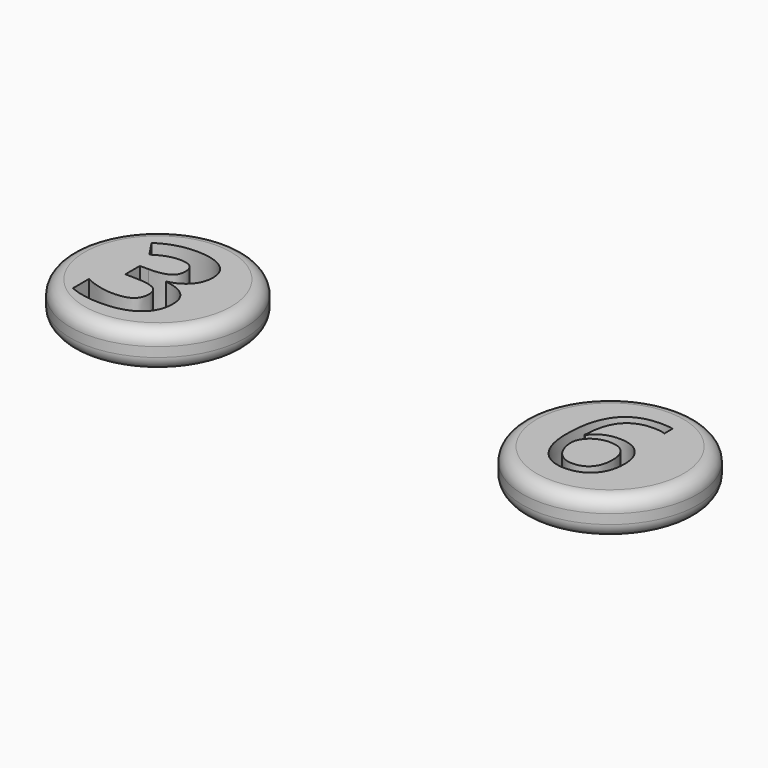
from build123d import *

# Parameters (mm, degrees)
F0_R         = 15.498811994
F1_DEPTH     = 6.604
F2_R         = 2.4528409794
F4_TEXT_SIZE = 27.8857070194
F5_DEPTH     = 25.4
F7_TEXT_SIZE = 25.6220861855
F8_DEPTH     = 25.4


# Not quite as in the source:
# - Text() gives the source's letters only with a copy of the font that has no kerning and outlines rounded to 1/6400 em; it was checked with that copy


with BuildPart() as f1:
    # F0 (on Top) → F1 (new body)
    with BuildSketch(Plane.XY):
        with Locations((-40.1489026845, 21.7293333262)):
            Circle(F0_R)
    extrude(amount=F1_DEPTH)

    # F2
    f2_edges = [f1.edges().sort_by_distance(p)[0] for p in [
        (-55.647715, 21.729333, 0),
        (-55.647715, 21.729333, 6.604),
    ]]
    fillet(f2_edges, radius=F2_R)


with BuildPart() as f3_1:
    # F3: instance of F1
    add(f1.part.mirror(Plane.YZ))

    # F7 (on face) → F8 (cut)
    with BuildSketch(Plane.XY.offset(6.604)):
        with Locations((31.6101685166, 12.9549875855)):
            Text('6', F7_TEXT_SIZE, font='Open Sans', text_align=(TextAlign.LEFT, TextAlign.BOTTOM))
    extrude(amount=-F8_DEPTH, mode=Mode.SUBTRACT)


with BuildPart() as f1_1:
    add(f1.part)

    # F4 (on face) → F5 (cut)
    with BuildSketch(Plane.XY.offset(6.604)):
        with Locations((-48.7448008959, 11.4652827976)):
            Text('3', F4_TEXT_SIZE, font='Open Sans', font_style=FontStyle.BOLD, text_align=(TextAlign.LEFT, TextAlign.BOTTOM))
    extrude(amount=-F5_DEPTH, mode=Mode.SUBTRACT)


solid = Compound([f3_1.part, f1_1.part])
